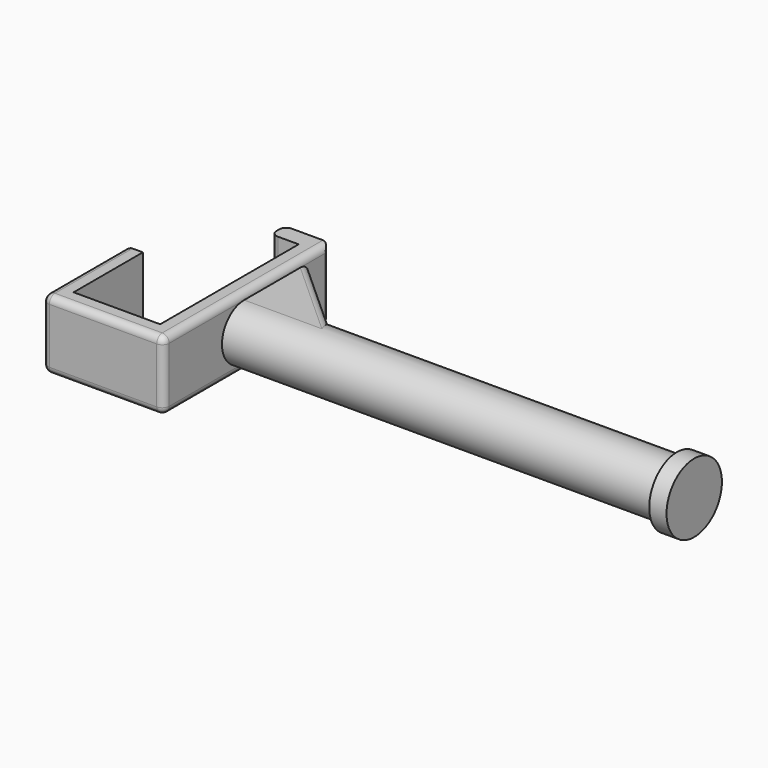
from build123d import *

# Parameters (mm, degrees)
F1_DEPTH     = 10
F2_R         = 8
F3_DEPTH     = 125
F4_R         = 10
F4_R_2       = 8
F5_DEPTH     = 5
F7_DEPTH     = 8
F8_T4_DEPTH  = 47.7749887628
F8_S5_R      = 8
F8_T6_DEPTH  = 26
F8_T11_DEPTH = 47.7749887628
F8_S12_R     = 8
F8_T13_DEPTH = 26
F9_R         = 1.99999


# Not quite as in the source:
# - a fillet or chamfer that OpenCascade refuses, or shapes differently, is made with other operations: its cross-section is extruded or revolved along the edge and cut away or added
# - a fillet or chamfer is up to 0.001 mm smaller than in the source, because OpenCascade refuses the exact size


with BuildPart() as f1:
    # F0 (on Top) → F1 (new body, symmetric)
    with BuildSketch(Plane.XY):
        Polygon((-33.2763881331, -24.0594327205), (-33.2763881331, 0.9405672795), (-38.2763881331, 0.9405672795), (-38.2763881331, -29.0594327205), (-3.2763881331, -29.0594327205), (-3.2763881331, 30.9405672795), (-16.2763881331, 30.9405672795), (-16.2763881331, 25.9405672795), (-8.2763881331, 25.9405672795), (-8.2763881331, -24.0594327205), align=None)
    extrude(amount=F1_DEPTH, both=True)

    # F2 (on face) → F3 (join)
    with BuildSketch(Plane.YZ.offset(-3.2763881331)):
        Circle(F2_R)
    extrude(amount=F3_DEPTH)

    # F4 (on face) → F5 (join)
    with BuildSketch(Plane.YZ.offset(121.7236118669)):
        Circle(F4_R)
        Circle(F4_R_2, mode=Mode.SUBTRACT)
        Circle(F4_R_2)
    extrude(amount=F5_DEPTH)

    # F6 (on Top) → F7 (join, symmetric)
    with BuildSketch(Plane.XY):
        Polygon((22.1584475915, 0), (-4.7209444456, 24.2796987295), (-7.46962009, 0), align=None)
    extrude(amount=F7_DEPTH, both=True)

    # F8: fillet of radius 2 on 2 edges, made by hand


with BuildPart() as f8_tool2:
    # F8_s3 → F8_t4 (new body)
    with BuildSketch(Plane(origin=(18.5100171986, -16.719784452, 0), x_dir=(0, 0, 1), z_dir=(-0.742081519, 0.6703096442, 0))):
        with BuildLine():
            ThreePointArc((6, 14.8530211221), (7.4142135624, 14.2672346845), (8, 12.8530211221))
            Line((8, 12.8530211221), (8, 14.8530211221))
            Line((8, 14.8530211221), (6, 14.8530211221))
        make_face()
    extrude(amount=F8_T4_DEPTH)

    # F8_s5 → F8_t6 (cut, symmetric)
    with BuildSketch(Plane.YZ.offset(10.1)):
        Circle(F8_S5_R)
    extrude(amount=F8_T6_DEPTH, both=True, mode=Mode.SUBTRACT)

    split(bisect_by=Plane.YZ.offset(-3.2763881331), keep=Keep.TOP)


with BuildPart() as f1_1:
    add(f1.part)

    # F8_t1: cut F8_tool2
    add(f8_tool2.part, mode=Mode.SUBTRACT)


with BuildPart() as f8_tool9:
    # F8_s10 → F8_t11 (new body)
    with BuildSketch(Plane(origin=(18.5100171986, -16.719784452, 0), x_dir=(0, 0, 1), z_dir=(-0.742081519, 0.6703096442, 0))):
        with BuildLine():
            ThreePointArc((-6, 14.8530211221), (-7.4142135624, 14.2672346845), (-8, 12.8530211221))
            Line((-8, 12.8530211221), (-8, 14.8530211221))
            Line((-8, 14.8530211221), (-6, 14.8530211221))
        make_face()
    extrude(amount=F8_T11_DEPTH)

    # F8_s12 → F8_t13 (cut, symmetric)
    with BuildSketch(Plane.YZ.offset(10.1)):
        Circle(F8_S12_R)
    extrude(amount=F8_T13_DEPTH, both=True, mode=Mode.SUBTRACT)

    split(bisect_by=Plane.YZ.offset(-3.2763881331), keep=Keep.TOP)


with BuildPart() as f1_2:
    add(f1_1.part)

    # F8_t8: cut F8_tool9
    add(f8_tool9.part, mode=Mode.SUBTRACT)

    # F9 (radius 2 in the source; OpenCascade refuses exactly that, so slightly less here)
    f9_edges = [f1_2.edges().sort_by_distance(p)[0] for p in [
        (-3.276388, 0.940567, 10),
        (-3.276388, 0.940567, -10),
        (-20.776388, -29.059433, 10),
        (-20.776388, -29.059433, -10),
        (-38.276388, -14.059433, 10),
        (-38.276388, -14.059433, -10),
        (-38.276388, -29.059433, 0),
        (-38.276388, 0.940567, 0),
        (-3.276388, -29.059433, 0),
        (-3.276388, 30.940567, 0),
        (-16.276388, 30.940567, 0),
        (-16.276388, 25.940567, 0),
    ]]
    fillet(f9_edges, radius=F9_R)


solid = f1_2.part
